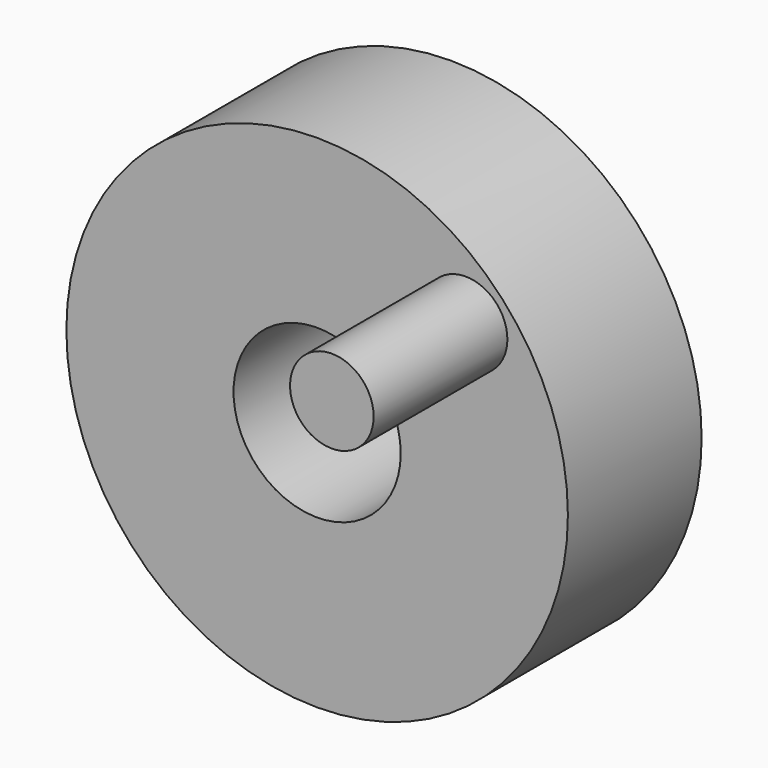
from build123d import *

# Parameters (mm, degrees)
F0_R     = 38.1
F0_R_2   = 12.7
F1_DEPTH = 12.7
F2_R     = 6.35
F3_DEPTH = 25.4


# Not quite as in the source:
# - a feature names something its author has since deleted; it is built from what else it names


with BuildPart() as f1:
    # F0 (on Front) → F1 (new body, symmetric)
    with BuildSketch(Plane.XZ):
        Circle(F0_R)
        Circle(F0_R_2, mode=Mode.SUBTRACT)
    extrude(amount=F1_DEPTH, both=True)

    # F2 (on face) → F3 (join)
    with BuildSketch(Plane.XZ.offset(12.7)):
        with Locations((22.5570311415, 20.5358944896)):
            Circle(F2_R)
    extrude(amount=F3_DEPTH)


solid = f1.part
